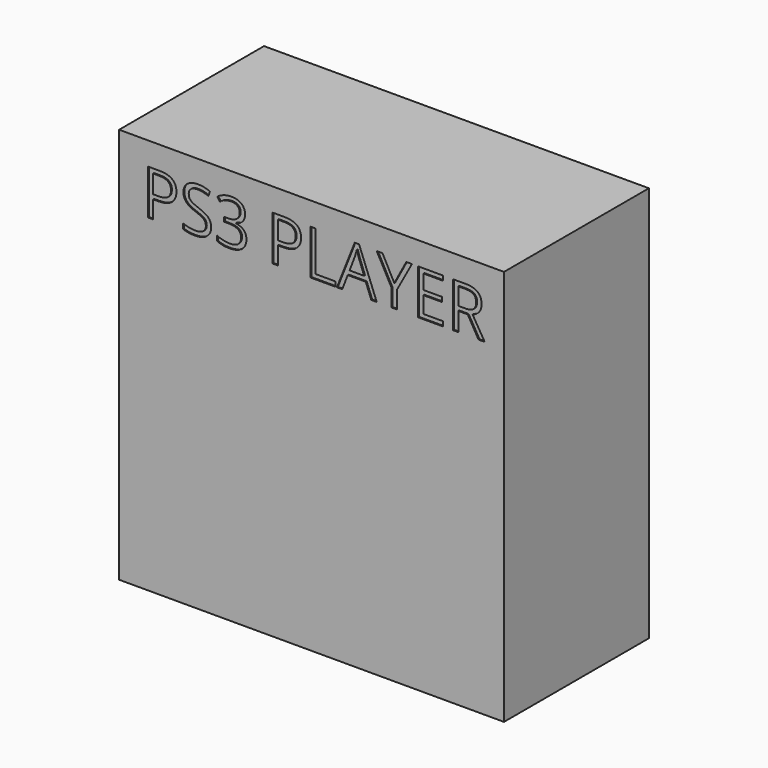
from build123d import *

# Parameters (mm, degrees)
F0_W         = 340
F0_H         = 160
F1_DEPTH     = 350
F2_TEXT_SIZE = 55.5555555556
F3_DEPTH     = 1


# Not quite as in the source:
# - Text() gives the source's letters only with a copy of the font that has no kerning and outlines rounded to 1/6400 em; it was checked with that copy


with BuildPart() as f1:
    # F0 (on Top) → F1 (new body)
    with BuildSketch(Plane.XY):
        Rectangle(F0_W, F0_H)
    extrude(amount=F1_DEPTH)

    # F2 (on face) → F3 (cut)
    with BuildSketch(Plane.XZ.offset(80)):
        with Locations((-150, 290)):
            Text('PS3 PLAYER', F2_TEXT_SIZE, font='Open Sans', text_align=(TextAlign.LEFT, TextAlign.BOTTOM))
    extrude(amount=-F3_DEPTH, mode=Mode.SUBTRACT)


solid = f1.part
